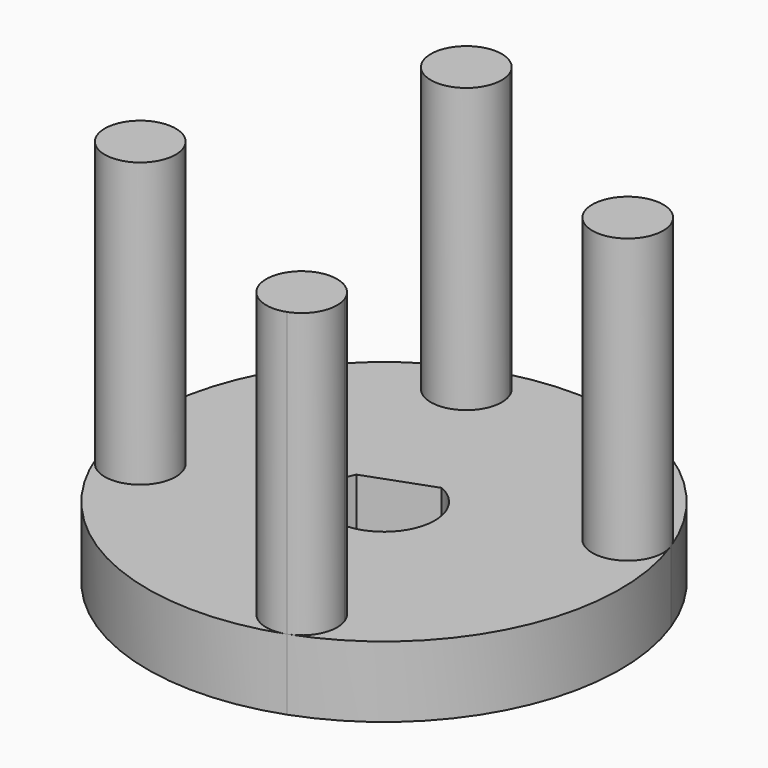
from build123d import *

# Parameters (mm, degrees)
F0_R     = 1.5
F1_DEPTH = 3
F2_DEPTH = 15
F4_ANGLE = 20


# Not quite as in the source:
# - a feature names something its author has since deleted; it is built from what else it names


with BuildPart() as f1:
    # F0 (on Top) → F1 (new body)
    with BuildSketch(Plane.XY):
        with BuildLine():
            ThreePointArc((4.3e-09, -10), (7.0710678134, -7.0710678103), (10, 0))
            ThreePointArc((10, 0), (7.0710678119, 7.0710678119), (0, 10))
            ThreePointArc((0, 10), (-7.0710678074, 7.0710678163), (-10, 1.26e-08))
            ThreePointArc((-10, 1.26e-08), (-7.0710678148, -7.0710678089), (4.3e-09, -10))
        make_face()
        with BuildLine():
            ThreePointArc((1.5, -8.5), (1.0606601733, -9.5606601703), (4.3e-09, -10))
            ThreePointArc((4.3e-09, -10), (-1.0606601733, -7.4393398297), (1.5, -8.5))
        make_face(mode=Mode.SUBTRACT)
        with BuildLine():
            ThreePointArc((-7, 0), (-8.5000000063, -1.5), (-10, 1.26e-08))
            ThreePointArc((-10, 1.26e-08), (-8.4999999937, 1.5), (-7, 0))
        make_face(mode=Mode.SUBTRACT)
        with BuildLine():
            ThreePointArc((1.4899664426, 1.55), (1.9781213122, 0.842339643), (2.15, 0))
            ThreePointArc((2.15, 0), (-0.842339643, -1.9781213122), (-1.4899664426, 1.55))
            ThreePointArc((-1.4899664426, 1.55), (0, 2.15), (1.4899664426, 1.55))
        make_face(mode=Mode.SUBTRACT)
        with Locations((8.5, 0)):
            Circle(F0_R, mode=Mode.SUBTRACT)
        with BuildLine():
            ThreePointArc((1.5, 8.5), (-1.0606601718, 7.4393398282), (0, 10))
            ThreePointArc((0, 10), (1.0606601718, 9.5606601718), (1.5, 8.5))
        make_face(mode=Mode.SUBTRACT)
        with BuildLine():
            ThreePointArc((-7, 0), (-8.4999999937, 1.5), (-10, 1.26e-08))
            ThreePointArc((-10, 1.26e-08), (-8.5000000063, -1.5), (-7, 0))
        make_face()
        with BuildLine():
            ThreePointArc((1.5, -8.5), (-1.0606601733, -7.4393398297), (4.3e-09, -10))
            ThreePointArc((4.3e-09, -10), (1.0606601733, -9.5606601703), (1.5, -8.5))
        make_face()
        with Locations((8.5, 0)):
            Circle(F0_R)
        with BuildLine():
            ThreePointArc((1.5, 8.5), (1.0606601718, 9.5606601718), (0, 10))
            ThreePointArc((0, 10), (-1.0606601718, 7.4393398282), (1.5, 8.5))
        make_face()
        with BuildLine():
            Line((-1.4899664426, 1.55), (1.4899664426, 1.55))
            ThreePointArc((1.4899664426, 1.55), (0, 2.15), (-1.4899664426, 1.55))
        make_face()
    extrude(amount=F1_DEPTH)

    # F0 (on Top) → F2 (join)
    with BuildSketch(Plane.XY):
        with BuildLine():
            ThreePointArc((1.5, 8.5), (1.0606601718, 9.5606601718), (0, 10))
            ThreePointArc((0, 10), (-1.0606601718, 7.4393398282), (1.5, 8.5))
        make_face()
        with BuildLine():
            ThreePointArc((-7, 0), (-8.4999999937, 1.5), (-10, 1.26e-08))
            ThreePointArc((-10, 1.26e-08), (-8.5000000063, -1.5), (-7, 0))
        make_face()
        with BuildLine():
            ThreePointArc((1.5, -8.5), (-1.0606601733, -7.4393398297), (4.3e-09, -10))
            ThreePointArc((4.3e-09, -10), (1.0606601733, -9.5606601703), (1.5, -8.5))
        make_face()
        with Locations((8.5, 0)):
            Circle(F0_R)
    extrude(amount=F2_DEPTH)


with BuildPart() as f1_1:
    # F4: moved
    add(f1.part.rotate(Axis((0, 0, 24.3583247066), (0, 0, 1)), F4_ANGLE))


solid = f1_1.part
